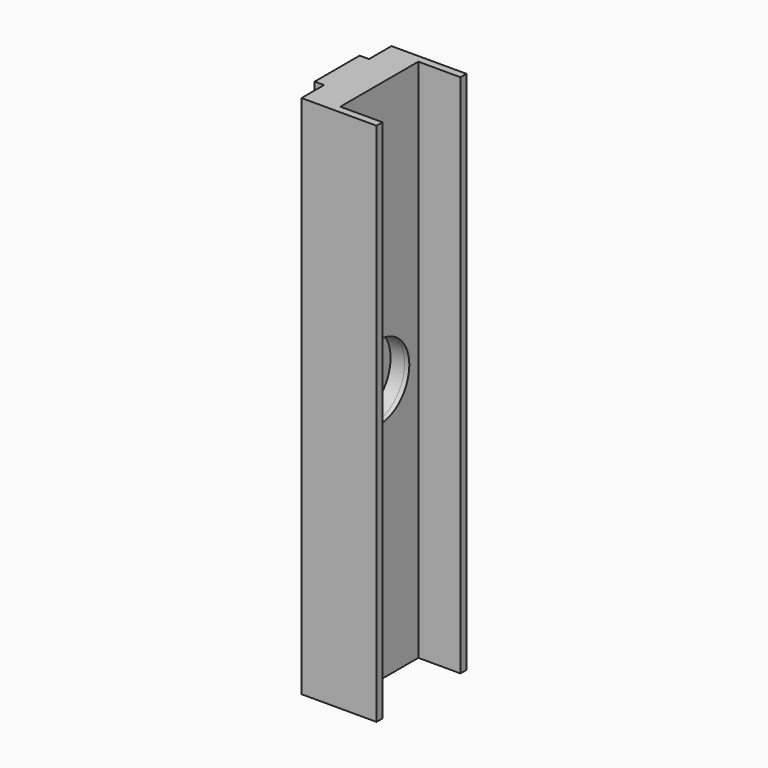
from build123d import *

# Parameters (mm, degrees)
F0_W           = 8
F0_H           = 12
F1_DEPTH       = 56
F2_W           = 5
F2_H           = 10.4
F3_DEPTH       = 56
F5_DEPTH       = 56
F7_D           = 5
F7_DEPTH       = 34
F7_CBORE_D     = 8
F7_CBORE_DEPTH = 1.5
F7_TIP         = 1.5021515476
F8_DEPTH       = 0.5


with BuildPart() as f1:
    # F0 (on Top) → F1 (new body)
    with BuildSketch(Plane.XY):
        with Locations((-63.4363747239, 8.6988127381)):
            Rectangle(F0_W, F0_H)
    extrude(amount=F1_DEPTH)

    # F2 (on face) → F3 (cut)
    with BuildSketch(Plane.XY.offset(56)):
        with Locations((-61.9363747239, 8.6988127381)):
            Rectangle(F2_W, F2_H)
    extrude(amount=-F3_DEPTH, mode=Mode.SUBTRACT)

    # F4 (on face) → F5 (join)
    with BuildSketch(Plane.XY.offset(56)):
        Polygon((-67.4363747239, 5.6988127381), (-67.4363747239, 8.6988127381), (-67.4363747239, 11.6988127381), (-68.4363747239, 11.6988127381), (-68.4363747239, 5.6988127381), align=None)
    extrude(amount=-F5_DEPTH)

    # F7
    with Locations(Plane.YZ.offset(-64.4363747239)):
        with Locations((8.6988127381, 28)):
            CounterBoreHole(F7_D / 2, F7_CBORE_D / 2, F7_CBORE_DEPTH, depth=F7_DEPTH)
            with Locations((0, 0, -(F7_DEPTH + F7_TIP / 2))):  # 118° drill point
                Cone(0, F7_D / 2, F7_TIP, mode=Mode.SUBTRACT)

    # F8 (add): a face of the model
    f8_faces = [f1.faces().sort_by_distance(p)[0] for p in [
        (-64.4363747239, 13.3292374577, 28),
    ]]
    extrude(f8_faces, amount=F8_DEPTH)


solid = f1.part
